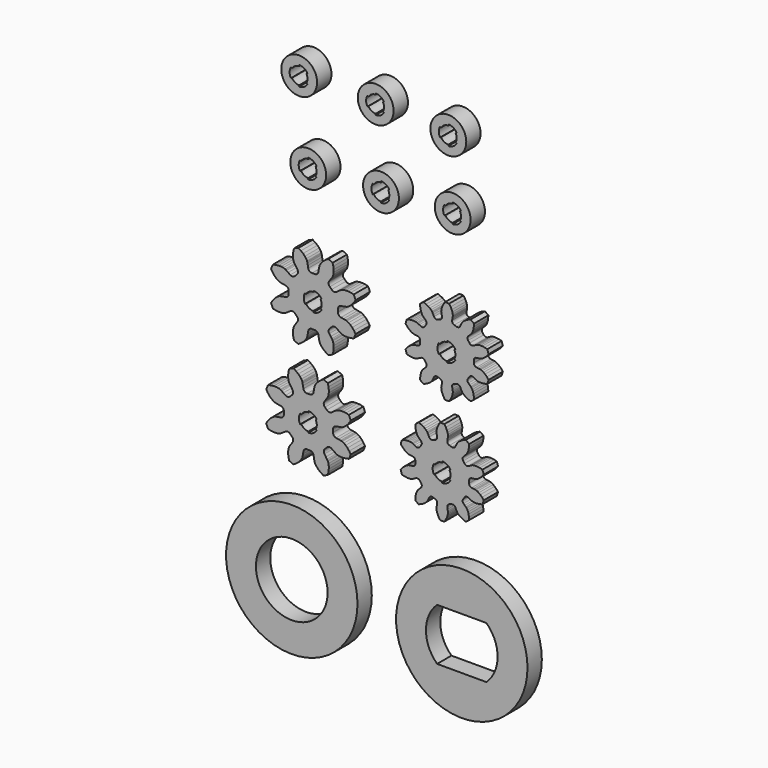
from build123d import *

# Parameters (mm, degrees)
F0_R     = 3
F1_DEPTH = 3
F0_R_2   = 11
F0_R_3   = 6


# Not quite as in the source:
# - ends of sketch curves that miss each other by under 0.0002 mm in the source are joined


with BuildPart() as f1:
    # F0 (on Front) → F1 (new body)
    with BuildSketch(Plane.XZ):
        with Locations((-0.182733, 41.3726)):
            Circle(F0_R)
        with BuildLine():
            ThreePointArc((-1.5683737345, 40.5726001533), (-1.782733, 41.3726), (-1.5683737345, 42.1725998467))
            Line((-1.5683737345, 42.1725998467), (-1.395169, 42.0726))
            ThreePointArc((-1.395169, 42.0726), (-0.8827330941, 42.585035511), (-0.182733, 42.7726))
            Line((-0.182733, 42.7726), (-0.182733, 42.9726))
            ThreePointArc((-0.182733, 42.9726), (0.6172670766, 42.7582406018), (1.2029077345, 42.1725998467))
            Line((1.2029077345, 42.1725998467), (1.029702, 42.0726))
            ThreePointArc((1.029702, 42.0726), (1.217267, 41.3726), (1.029702424, 40.6725997552))
            Line((1.029702424, 40.6725997552), (1.202908, 40.5726))
            ThreePointArc((1.202908, 40.5726), (0.6172670766, 39.9869593982), (-0.182733, 39.7726))
            Line((-0.182733, 39.7726), (-0.182733, 39.9726))
            ThreePointArc((-0.182733, 39.9726), (-0.8827330941, 40.160164489), (-1.395168674, 40.6726001882))
            Line((-1.395168674, 40.6726001882), (-1.5683737345, 40.5726001533))
        make_face(mode=Mode.SUBTRACT)
    extrude(amount=F1_DEPTH)


with BuildPart() as f1b:
    # F0 (on Front) → F1, piece 2 (new body)
    with BuildSketch(Plane.XZ):
        with Locations((12.707934, 29.490534)):
            Circle(F0_R)
        with BuildLine():
            ThreePointArc((11.3222932655, 28.6905341533), (11.107934, 29.490534), (11.3222932655, 30.2905338467))
            Line((11.3222932655, 30.2905338467), (11.495498, 30.190534))
            ThreePointArc((11.495498, 30.190534), (12.0079339059, 30.702969511), (12.707934, 30.890534))
            Line((12.707934, 30.890534), (12.707934, 31.090534))
            ThreePointArc((12.707934, 31.090534), (13.5079338601, 30.8761747268), (14.0935744845, 30.2905342798))
            Line((14.0935744845, 30.2905342798), (13.920369, 30.190534))
            ThreePointArc((13.920369, 30.190534), (14.107934, 29.490534), (13.920369424, 28.7905337552))
            Line((13.920369424, 28.7905337552), (14.093574, 28.690534))
            ThreePointArc((14.093574, 28.690534), (13.5079338601, 28.1048932732), (12.707934, 27.890534))
            Line((12.707934, 27.890534), (12.707934, 28.090534))
            ThreePointArc((12.707934, 28.090534), (12.0079339059, 28.278098489), (11.495498326, 28.7905341882))
            Line((11.495498326, 28.7905341882), (11.3222932655, 28.6905341533))
        make_face(mode=Mode.SUBTRACT)
    extrude(amount=F1_DEPTH)


with BuildPart() as f1c:
    # F0 (on Front) → F1, piece 3 (new body)
    with BuildSketch(Plane.XZ):
        with Locations((14.22888, -33.401225)):
            Circle(F0_R_2)
        with BuildLine():
            ThreePointArc((10.1003209518, -37.7549590508), (8.22888, -33.401225), (10.1003209518, -29.0474909492))
            Line((10.100321, -29.047491), (18.357439, -29.047491))
            ThreePointArc((18.3574390482, -29.0474909492), (20.22888, -33.401225), (18.3574390482, -37.7549590508))
            Line((18.357439, -37.754959), (10.100321, -37.754959))
        make_face(mode=Mode.SUBTRACT)
    extrude(amount=F1_DEPTH)


with BuildPart() as f1d:
    # F0 (on Front) → F1, piece 4 (new body)
    with BuildSketch(Plane.XZ):
        with BuildLine():
            ThreePointArc((13.143043773, -4.7593788891), (12.8821829065, -5.001442346), (12.5263362927, -5.0054792153))
            ThreePointArc((12.5263362927, -5.0054792153), (12.3443007022, -4.9419897506), (12.1597130423, -4.8863558479))
            ThreePointArc((12.1597130423, -4.8863558479), (11.8741990901, -4.6739288738), (11.8054388864, -4.32476498))
            Line((11.8054388864, -4.32476498), (11.855269, -4.040146))
            Line((11.855269, -4.040146), (11.893883, -3.81665))
            Line((11.893883, -3.81665), (11.91335, -3.700308))
            Line((11.91335, -3.700308), (11.920983, -3.648286))
            Line((11.920983, -3.648286), (11.923445, -3.579347))
            Line((11.923445, -3.579347), (11.903044, -3.355628))
            Line((11.903044, -3.355628), (11.840028, -3.082864))
            Line((11.840028, -3.082864), (11.732643, -2.782696))
            Line((11.732643, -2.782696), (11.549308, -2.410137))
            Line((11.549308, -2.410137), (11.30583, -2.030359))
            ThreePointArc((11.30583, -2.030359), (10.953724, -2.021744), (10.6016179893, -2.0303587818))
            Line((10.6016179893, -2.0303587818), (10.35814, -2.410137))
            Line((10.35814, -2.410137), (10.174805, -2.782696))
            Line((10.174805, -2.782696), (10.06742, -3.082864))
            Line((10.06742, -3.082864), (10.004404, -3.355628))
            Line((10.004404, -3.355628), (9.984003, -3.579347))
            Line((9.984003, -3.579347), (9.986465, -3.648286))
            Line((9.986465, -3.648286), (9.994098, -3.700308))
            Line((9.994098, -3.700308), (10.013565, -3.81665))
            Line((10.013565, -3.81665), (10.052179, -4.040146))
            Line((10.052179, -4.040146), (10.102009, -4.324765))
            ThreePointArc((10.102009, -4.324765), (10.0332489099, -4.6739288738), (9.7477349098, -4.8863556756))
            ThreePointArc((9.7477349098, -4.8863556756), (9.5631472978, -4.9419897506), (9.3811119632, -5.0054789014))
            ThreePointArc((9.3811119632, -5.0054789014), (9.0252650935, -5.001442346), (8.764404227, -4.7593788891))
            Line((8.764404227, -4.7593788891), (8.637422, -4.499829))
            Line((8.637422, -4.499829), (8.537294, -4.296319))
            Line((8.537294, -4.296319), (8.484659, -4.190755))
            Line((8.484659, -4.190755), (8.460257, -4.144181))
            Line((8.460257, -4.144181), (8.421727, -4.086962))
            Line((8.421727, -4.086962), (8.273723, -3.91796))
            Line((8.273723, -3.91796), (8.062416, -3.734329))
            Line((8.062416, -3.734329), (7.799105, -3.554608))
            Line((7.799105, -3.554608), (7.431799, -3.360962))
            Line((7.431799, -3.360962), (7.011593, -3.196829))
            ThreePointArc((7.011593, -3.196829), (6.7216698038, -3.3968219164), (6.4418739653, -3.6107539568))
            Line((6.4418739653, -3.6107539568), (6.468124, -4.061113))
            Line((6.468124, -4.061113), (6.538788, -4.470281))
            Line((6.538788, -4.470281), (6.628346, -4.776242))
            Line((6.628346, -4.776242), (6.737691, -5.033952))
            Line((6.737691, -5.033952), (6.852686, -5.226936))
            Line((6.852686, -5.226936), (6.895199, -5.281263))
            Line((6.895199, -5.281263), (6.931952, -5.318862))
            Line((6.931952, -5.318862), (7.016084, -5.401543))
            Line((7.016084, -5.401543), (7.178692, -5.559658))
            Line((7.178692, -5.559658), (7.3863, -5.76063))
            ThreePointArc((7.3863, -5.76063), (7.535905329, -6.0835261569), (7.4297816373, -6.423203712))
            ThreePointArc((7.4297816373, -6.423203712), (7.3131475737, -6.5767102981), (7.2031958069, -6.7350718719))
            ThreePointArc((7.2031958069, -6.7350718719), (6.912937393, -6.9409680096), (6.5596149724, -6.8984650521))
            Line((6.5596149724, -6.8984650521), (6.304324, -6.763122))
            Line((6.304324, -6.763122), (6.103699, -6.657333))
            Line((6.103699, -6.657333), (5.999067, -6.602868))
            Line((5.999067, -6.602868), (5.95195, -6.579533))
            Line((5.95195, -6.579533), (5.887146, -6.555888))
            Line((5.887146, -6.555888), (5.668072, -6.506157))
            Line((5.668072, -6.506157), (5.389185, -6.4818))
            Line((5.389185, -6.4818), (5.070524, -6.491173))
            Line((5.070524, -6.491173), (4.659546, -6.550407))
            Line((4.659546, -6.550407), (4.223117, -6.664611))
            ThreePointArc((4.223117, -6.664611), (4.106117181, -6.996821338), (4.0055036402, -7.3343559023))
            Line((4.0055036402, -7.3343559023), (4.291455, -7.683276))
            Line((4.291455, -7.683276), (4.589126, -7.972764))
            Line((4.589126, -7.972764), (4.841419, -8.167651))
            Line((4.841419, -8.167651), (5.08136, -8.311871))
            Line((5.08136, -8.311871), (5.287825, -8.400406))
            Line((5.287825, -8.400406), (5.354151, -8.419369))
            Line((5.354151, -8.419369), (5.405986, -8.428185))
            Line((5.405986, -8.428185), (5.522649, -8.445623))
            Line((5.522649, -8.445623), (5.747139, -8.477962))
            Line((5.747139, -8.477962), (6.033226, -8.518523))
            ThreePointArc((6.033226, -8.518523), (6.3440523322, -8.6918157461), (6.4578534569, -9.0289989767))
            ThreePointArc((6.4578534569, -9.0289989767), (6.453724, -9.221744), (6.4578537438, -9.414489011))
            ThreePointArc((6.4578537438, -9.414489011), (6.3440522875, -9.7516723076), (6.0332259646, -9.9249647496))
            Line((6.0332259646, -9.9249647496), (5.747139, -9.965526))
            Line((5.747139, -9.965526), (5.522649, -9.997865))
            Line((5.522649, -9.997865), (5.405986, -10.015303))
            Line((5.405986, -10.015303), (5.354151, -10.024119))
            Line((5.354151, -10.024119), (5.287825, -10.043082))
            Line((5.287825, -10.043082), (5.08136, -10.131617))
            Line((5.08136, -10.131617), (4.841419, -10.275837))
            Line((4.841419, -10.275837), (4.589126, -10.470724))
            Line((4.589126, -10.470724), (4.291455, -10.760212))
            Line((4.291455, -10.760212), (4.005504, -11.109132))
            ThreePointArc((4.005504, -11.109132), (4.1061173301, -11.4466671209), (4.2231169849, -11.7788770057))
            Line((4.2231169849, -11.7788770057), (4.659546, -11.893081))
            Line((4.659546, -11.893081), (5.070524, -11.952315))
            Line((5.070524, -11.952315), (5.389185, -11.961688))
            Line((5.389185, -11.961688), (5.668072, -11.937331))
            Line((5.668072, -11.937331), (5.887146, -11.8876))
            Line((5.887146, -11.8876), (5.95195, -11.863955))
            Line((5.95195, -11.863955), (5.999067, -11.84062))
            Line((5.999067, -11.84062), (6.103699, -11.786155))
            Line((6.103699, -11.786155), (6.304324, -11.680366))
            Line((6.304324, -11.680366), (6.559615, -11.545023))
            ThreePointArc((6.559615, -11.545023), (6.912937393, -11.5025199904), (7.2031960279, -11.7084159815))
            ThreePointArc((7.2031960279, -11.7084159815), (7.3131480487, -11.8667783558), (7.4297819085, -12.0202850727))
            ThreePointArc((7.4297819085, -12.0202850727), (7.5359052806, -12.3599625806), (7.3862996155, -12.6828576024))
            Line((7.3862996155, -12.6828576024), (7.178692, -12.88383))
            Line((7.178692, -12.88383), (7.016084, -13.041945))
            Line((7.016084, -13.041945), (6.931952, -13.124626))
            Line((6.931952, -13.124626), (6.895199, -13.162225))
            Line((6.895199, -13.162225), (6.852686, -13.216552))
            Line((6.852686, -13.216552), (6.737691, -13.409536))
            Line((6.737691, -13.409536), (6.628346, -13.667246))
            Line((6.628346, -13.667246), (6.538788, -13.973207))
            Line((6.538788, -13.973207), (6.468124, -14.382375))
            Line((6.468124, -14.382375), (6.441874, -14.832734))
            ThreePointArc((6.441874, -14.832734), (6.7216700253, -15.0466662445), (7.0115933661, -15.2466594405))
            Line((7.0115933661, -15.2466594405), (7.431799, -15.082526))
            Line((7.431799, -15.082526), (7.799105, -14.88888))
            Line((7.799105, -14.88888), (8.062416, -14.709159))
            Line((8.062416, -14.709159), (8.273723, -14.525528))
            Line((8.273723, -14.525528), (8.421727, -14.356526))
            Line((8.421727, -14.356526), (8.460257, -14.299307))
            Line((8.460257, -14.299307), (8.484659, -14.252733))
            Line((8.484659, -14.252733), (8.537294, -14.147169))
            Line((8.537294, -14.147169), (8.637422, -13.943659))
            Line((8.637422, -13.943659), (8.764404, -13.684109))
            ThreePointArc((8.764404, -13.684109), (9.0252648386, -13.4420457557), (9.3811120348, -13.4380089068))
            ThreePointArc((9.3811120348, -13.4380089068), (9.5631475914, -13.5014983448), (9.7477352159, -13.557132224))
            ThreePointArc((9.7477352159, -13.557132224), (10.0332489814, -13.7695592395), (10.1020091136, -14.11872302))
            Line((10.1020091136, -14.11872302), (10.052179, -14.403342))
            Line((10.052179, -14.403342), (10.013565, -14.626838))
            Line((10.013565, -14.626838), (9.994098, -14.74318))
            Line((9.994098, -14.74318), (9.986465, -14.795202))
            Line((9.986465, -14.795202), (9.984003, -14.864141))
            Line((9.984003, -14.864141), (10.004404, -15.08786))
            Line((10.004404, -15.08786), (10.06742, -15.360624))
            Line((10.06742, -15.360624), (10.174805, -15.660792))
            Line((10.174805, -15.660792), (10.35814, -16.033351))
            Line((10.35814, -16.033351), (10.601618, -16.413129))
            ThreePointArc((10.601618, -16.413129), (10.953724, -16.421744), (11.3058299618, -16.4131292206))
            Line((11.3058299618, -16.4131292206), (11.549308, -16.033351))
            Line((11.549308, -16.033351), (11.732643, -15.660792))
            Line((11.732643, -15.660792), (11.840028, -15.360624))
            Line((11.840028, -15.360624), (11.903044, -15.08786))
            Line((11.903044, -15.08786), (11.923445, -14.864141))
            Line((11.923445, -14.864141), (11.920983, -14.795202))
            Line((11.920983, -14.795202), (11.91335, -14.74318))
            Line((11.91335, -14.74318), (11.893883, -14.626838))
            Line((11.893883, -14.626838), (11.855269, -14.403342))
            Line((11.855269, -14.403342), (11.805439, -14.118723))
            ThreePointArc((11.805439, -14.118723), (11.8741990186, -13.7695592395), (12.159712832, -13.5571323962))
            ThreePointArc((12.159712832, -13.5571323962), (12.3443004086, -13.5014983448), (12.5263357093, -13.4380092207))
            ThreePointArc((12.5263357093, -13.4380092207), (12.8821831614, -13.4420457557), (13.1430441674, -13.6841099182))
            Line((13.1430441674, -13.6841099182), (13.270026, -13.943659))
            Line((13.270026, -13.943659), (13.370154, -14.147169))
            Line((13.370154, -14.147169), (13.422789, -14.252733))
            Line((13.422789, -14.252733), (13.447191, -14.299307))
            Line((13.447191, -14.299307), (13.485721, -14.356526))
            Line((13.485721, -14.356526), (13.633725, -14.525528))
            Line((13.633725, -14.525528), (13.845032, -14.709159))
            Line((13.845032, -14.709159), (14.108343, -14.88888))
            Line((14.108343, -14.88888), (14.475649, -15.082526))
            Line((14.475649, -15.082526), (14.895855, -15.246659))
            ThreePointArc((14.895855, -15.246659), (15.1857779747, -15.0466662445), (15.4655740347, -14.8327340432))
            Line((15.4655740347, -14.8327340432), (15.439324, -14.382375))
            Line((15.439324, -14.382375), (15.36866, -13.973207))
            Line((15.36866, -13.973207), (15.279102, -13.667246))
            Line((15.279102, -13.667246), (15.169757, -13.409536))
            Line((15.169757, -13.409536), (15.054762, -13.216552))
            Line((15.054762, -13.216552), (15.012249, -13.162225))
            Line((15.012249, -13.162225), (14.975496, -13.124626))
            Line((14.975496, -13.124626), (14.891364, -13.041945))
            Line((14.891364, -13.041945), (14.728756, -12.88383))
            Line((14.728756, -12.88383), (14.521148, -12.682858))
            ThreePointArc((14.521148, -12.682858), (14.3715427226, -12.359962629), (14.4776662624, -12.0202844143))
            ThreePointArc((14.4776662624, -12.0202844143), (14.594300134, -11.8667781042), (14.7042517326, -11.7084168227))
            ThreePointArc((14.7042517326, -11.7084168227), (14.994510607, -11.5025199904), (15.3478330276, -11.5450229479))
            Line((15.3478330276, -11.5450229479), (15.603124, -11.680366))
            Line((15.603124, -11.680366), (15.803749, -11.786155))
            Line((15.803749, -11.786155), (15.908381, -11.84062))
            Line((15.908381, -11.84062), (15.955498, -11.863955))
            Line((15.955498, -11.863955), (16.020302, -11.8876))
            Line((16.020302, -11.8876), (16.239376, -11.937331))
            Line((16.239376, -11.937331), (16.518263, -11.961688))
            Line((16.518263, -11.961688), (16.836924, -11.952315))
            Line((16.836924, -11.952315), (17.247902, -11.893081))
            Line((17.247902, -11.893081), (17.684331, -11.778877))
            ThreePointArc((17.684331, -11.778877), (17.8013307104, -11.4466669962), (17.9019441756, -11.1091327761))
            Line((17.9019441756, -11.1091327761), (17.615993, -10.760212))
            Line((17.615993, -10.760212), (17.318322, -10.470724))
            Line((17.318322, -10.470724), (17.066029, -10.275837))
            Line((17.066029, -10.275837), (16.826088, -10.131617))
            Line((16.826088, -10.131617), (16.619623, -10.043082))
            Line((16.619623, -10.043082), (16.553297, -10.024119))
            Line((16.553297, -10.024119), (16.501462, -10.015303))
            Line((16.501462, -10.015303), (16.384799, -9.997865))
            Line((16.384799, -9.997865), (16.160309, -9.965526))
            Line((16.160309, -9.965526), (15.874222, -9.924965))
            ThreePointArc((15.874222, -9.924965), (15.5633956988, -9.7516722911), (15.4495945449, -9.4144889805))
            ThreePointArc((15.4495945449, -9.4144889805), (15.453724, -9.221744), (15.4495942581, -9.0289990318))
            ThreePointArc((15.4495942581, -9.0289990318), (15.5633956541, -8.6918157626), (15.8742218969, -8.51852327))
            Line((15.8742218969, -8.51852327), (16.160309, -8.477962))
            Line((16.160309, -8.477962), (16.384799, -8.445623))
            Line((16.384799, -8.445623), (16.501462, -8.428185))
            Line((16.501462, -8.428185), (16.553297, -8.419369))
            Line((16.553297, -8.419369), (16.619623, -8.400406))
            Line((16.619623, -8.400406), (16.826088, -8.311871))
            Line((16.826088, -8.311871), (17.066029, -8.167651))
            Line((17.066029, -8.167651), (17.318322, -7.972764))
            Line((17.318322, -7.972764), (17.615993, -7.683276))
            Line((17.615993, -7.683276), (17.901944, -7.334356))
            ThreePointArc((17.901944, -7.334356), (17.8013308596, -6.9968214627), (17.6843310151, -6.6646109943))
            Line((17.6843310151, -6.6646109943), (17.247902, -6.550407))
            Line((17.247902, -6.550407), (16.836924, -6.491173))
            Line((16.836924, -6.491173), (16.518263, -6.4818))
            Line((16.518263, -6.4818), (16.239376, -6.506157))
            Line((16.239376, -6.506157), (16.020302, -6.555888))
            Line((16.020302, -6.555888), (15.955498, -6.579533))
            Line((15.955498, -6.579533), (15.908381, -6.602868))
            Line((15.908381, -6.602868), (15.803749, -6.657333))
            Line((15.803749, -6.657333), (15.603124, -6.763122))
            Line((15.603124, -6.763122), (15.347833, -6.898465))
            ThreePointArc((15.347833, -6.898465), (14.994510607, -6.9409680096), (14.7042519721, -6.7350720185))
            ThreePointArc((14.7042519721, -6.7350720185), (14.5943006091, -6.5767105497), (14.4776669653, -6.4232040276))
            ThreePointArc((14.4776669653, -6.4232040276), (14.3715426742, -6.0835261085), (14.5211484016, -5.7606303811))
            Line((14.5211484016, -5.7606303811), (14.728756, -5.559658))
            Line((14.728756, -5.559658), (14.891364, -5.401543))
            Line((14.891364, -5.401543), (14.975496, -5.318862))
            Line((14.975496, -5.318862), (15.012249, -5.281263))
            Line((15.012249, -5.281263), (15.054762, -5.226936))
            Line((15.054762, -5.226936), (15.169757, -5.033952))
            Line((15.169757, -5.033952), (15.279102, -4.776242))
            Line((15.279102, -4.776242), (15.36866, -4.470281))
            Line((15.36866, -4.470281), (15.439324, -4.061113))
            Line((15.439324, -4.061113), (15.465574, -3.610754))
            ThreePointArc((15.465574, -3.610754), (15.1857781962, -3.3968219164), (14.8958550921, -3.1968288593))
            Line((14.8958550921, -3.1968288593), (14.475649, -3.360962))
            Line((14.475649, -3.360962), (14.108343, -3.554608))
            Line((14.108343, -3.554608), (13.845032, -3.734329))
            Line((13.845032, -3.734329), (13.633725, -3.91796))
            Line((13.633725, -3.91796), (13.485721, -4.086962))
            Line((13.485721, -4.086962), (13.447191, -4.144181))
            Line((13.447191, -4.144181), (13.422789, -4.190755))
            Line((13.422789, -4.190755), (13.370154, -4.296319))
            Line((13.370154, -4.296319), (13.270026, -4.499829))
            Line((13.270026, -4.499829), (13.143043773, -4.7593788891))
        make_face()
        with BuildLine():
            ThreePointArc((9.5680835155, -10.0217442798), (9.353724, -9.221744), (9.5680835155, -8.4217437202))
            Line((9.5680835155, -8.4217437202), (9.741289, -8.521744))
            ThreePointArc((9.741289, -8.521744), (10.2537241224, -8.009308364), (10.953724, -7.821744))
            Line((10.953724, -7.821744), (10.953724, -7.621744))
            ThreePointArc((10.953724, -7.621744), (11.7537240766, -7.8361033982), (12.3393647345, -8.4217441533))
            Line((12.3393647345, -8.4217441533), (12.16616, -8.521744))
            ThreePointArc((12.16616, -8.521744), (12.353724, -9.221744), (12.166159674, -9.9217438118))
            Line((12.166159674, -9.9217438118), (12.339365, -10.021744))
            ThreePointArc((12.339365, -10.021744), (11.7537240766, -10.6073846018), (10.953724, -10.821744))
            Line((10.953724, -10.821744), (10.953724, -10.621744))
            ThreePointArc((10.953724, -10.621744), (10.2537241224, -10.434179636), (9.741288576, -9.9217442448))
            Line((9.741288576, -9.9217442448), (9.5680835155, -10.0217442798))
        make_face(mode=Mode.SUBTRACT)
    extrude(amount=F1_DEPTH)


with BuildPart() as f1e:
    # F0 (on Front) → F1, piece 5 (new body)
    with BuildSketch(Plane.XZ):
        with Locations((11.978656, 40.770012)):
            Circle(F0_R)
        with BuildLine():
            ThreePointArc((10.5930152655, 39.9700121533), (10.378656, 40.770012), (10.5930152655, 41.5700118467))
            Line((10.5930152655, 41.5700118467), (10.76622, 41.470012))
            ThreePointArc((10.76622, 41.470012), (11.2786559059, 41.982447511), (11.978656, 42.170012))
            Line((11.978656, 42.170012), (11.978656, 42.370012))
            ThreePointArc((11.978656, 42.370012), (12.7786560766, 42.1556526018), (13.3642967345, 41.5700118467))
            Line((13.3642967345, 41.5700118467), (13.191091, 41.470012))
            ThreePointArc((13.191091, 41.470012), (13.378656, 40.770012), (13.191091424, 40.0700117552))
            Line((13.191091424, 40.0700117552), (13.364297, 39.970012))
            ThreePointArc((13.364297, 39.970012), (12.7786560766, 39.3843713982), (11.978656, 39.170012))
            Line((11.978656, 39.170012), (11.978656, 39.370012))
            ThreePointArc((11.978656, 39.370012), (11.2786559059, 39.557576489), (10.766220326, 40.0700121882))
            Line((10.766220326, 40.0700121882), (10.5930152655, 39.9700121533))
        make_face(mode=Mode.SUBTRACT)
    extrude(amount=F1_DEPTH)


with BuildPart() as f1f:
    # F0 (on Front) → F1, piece 6 (new body)
    with BuildSketch(Plane.XZ):
        with BuildLine():
            Line((-4.705382, 7.712101), (-4.96919, 7.850628))
            Line((-4.96919, 7.850628), (-5.016148, 7.86832))
            Line((-5.016148, 7.86832), (-5.054828, 7.880652))
            Line((-5.054828, 7.880652), (-5.110027, 7.892802))
            Line((-5.110027, 7.892802), (-5.267232, 7.922637))
            Line((-5.267232, 7.922637), (-5.590275, 7.98214))
            Line((-5.590275, 7.98214), (-6.009857, 8.058547))
            ThreePointArc((-6.009857, 8.058547), (-6.3758616121, 8.27828494), (-6.5052699472, 8.6850989972))
            ThreePointArc((-6.5052699472, 8.6850989972), (-6.49946, 8.903954), (-6.5052698508, 9.1228090079))
            ThreePointArc((-6.5052698508, 9.1228090079), (-6.3758615567, 9.5296231301), (-6.0098568574, 9.7493612146))
            Line((-6.0098568574, 9.7493612146), (-5.590275, 9.825768))
            Line((-5.590275, 9.825768), (-5.267232, 9.885271))
            Line((-5.267232, 9.885271), (-5.110027, 9.915106))
            Line((-5.110027, 9.915106), (-5.054828, 9.927256))
            Line((-5.054828, 9.927256), (-5.016148, 9.939588))
            Line((-5.016148, 9.939588), (-4.96919, 9.95728))
            Line((-4.96919, 9.95728), (-4.705382, 10.095807))
            Line((-4.705382, 10.095807), (-4.408211, 10.317379))
            Line((-4.408211, 10.317379), (-4.106544, 10.612691))
            Line((-4.106544, 10.612691), (-3.816783, 10.974283))
            Line((-3.816783, 10.974283), (-3.5505, 11.39576))
            ThreePointArc((-3.5505, 11.39576), (-3.6953636243, 11.7740800279), (-3.8604425516, 12.1440262148))
            Line((-3.8604425516, 12.1440262148), (-4.346761, 12.253765))
            Line((-4.346761, 12.253765), (-4.807338, 12.304557))
            Line((-4.807338, 12.304557), (-5.229466, 12.300063))
            Line((-5.229466, 12.300063), (-5.596273, 12.246607))
            Line((-5.596273, 12.246607), (-5.880766, 12.15802))
            Line((-5.880766, 12.15802), (-5.926481, 12.137326))
            Line((-5.926481, 12.137326), (-5.962552, 12.118695))
            Line((-5.962552, 12.118695), (-6.010175, 12.088254))
            Line((-6.010175, 12.088254), (-6.142432, 11.99819))
            Line((-6.142432, 11.99819), (-6.412932, 11.811839))
            Line((-6.412932, 11.811839), (-6.76365, 11.569178))
            ThreePointArc((-6.76365, 11.569178), (-7.177832399, 11.4657525161), (-7.5569989389, 11.6619080549))
            ThreePointArc((-7.5569989389, 11.6619080549), (-7.7076450269, 11.8207699717), (-7.8665072327, 11.9714157412))
            ThreePointArc((-7.8665072327, 11.9714157412), (-8.0626615328, 12.3505820196), (-7.9592357689, 12.7647638399))
            Line((-7.9592357689, 12.7647638399), (-7.716575, 13.115482))
            Line((-7.716575, 13.115482), (-7.530224, 13.385982))
            Line((-7.530224, 13.385982), (-7.44016, 13.518239))
            Line((-7.44016, 13.518239), (-7.409719, 13.565862))
            Line((-7.409719, 13.565862), (-7.391088, 13.601933))
            Line((-7.391088, 13.601933), (-7.370394, 13.647648))
            Line((-7.370394, 13.647648), (-7.281807, 13.932141))
            Line((-7.281807, 13.932141), (-7.228351, 14.298948))
            Line((-7.228351, 14.298948), (-7.223857, 14.721076))
            Line((-7.223857, 14.721076), (-7.274649, 15.181653))
            Line((-7.274649, 15.181653), (-7.384388, 15.667972))
            ThreePointArc((-7.384388, 15.667972), (-7.7543343252, 15.833050522), (-8.13265416, 15.9779135458))
            Line((-8.13265416, 15.9779135458), (-8.554131, 15.711631))
            Line((-8.554131, 15.711631), (-8.915723, 15.42187))
            Line((-8.915723, 15.42187), (-9.211035, 15.120203))
            Line((-9.211035, 15.120203), (-9.432607, 14.823032))
            Line((-9.432607, 14.823032), (-9.571134, 14.559224))
            Line((-9.571134, 14.559224), (-9.588826, 14.512266))
            Line((-9.588826, 14.512266), (-9.601158, 14.473586))
            Line((-9.601158, 14.473586), (-9.613308, 14.418387))
            Line((-9.613308, 14.418387), (-9.643143, 14.261182))
            Line((-9.643143, 14.261182), (-9.702646, 13.938139))
            Line((-9.702646, 13.938139), (-9.779053, 13.518557))
            ThreePointArc((-9.779053, 13.518557), (-9.9987909608, 13.1525523715), (-10.4056050502, 13.0231440556))
            ThreePointArc((-10.4056050502, 13.0231440556), (-10.62446, 13.028954), (-10.8433149549, 13.023144152))
            ThreePointArc((-10.8433149549, 13.023144152), (-11.2501290392, 13.1525523715), (-11.4698671826, 13.5185569668))
            Line((-11.4698671826, 13.5185569668), (-11.546274, 13.938139))
            Line((-11.546274, 13.938139), (-11.605777, 14.261182))
            Line((-11.605777, 14.261182), (-11.635612, 14.418387))
            Line((-11.635612, 14.418387), (-11.647762, 14.473586))
            Line((-11.647762, 14.473586), (-11.660094, 14.512266))
            Line((-11.660094, 14.512266), (-11.677786, 14.559224))
            Line((-11.677786, 14.559224), (-11.816313, 14.823032))
            Line((-11.816313, 14.823032), (-12.037885, 15.120203))
            Line((-12.037885, 15.120203), (-12.333197, 15.42187))
            Line((-12.333197, 15.42187), (-12.694789, 15.711631))
            Line((-12.694789, 15.711631), (-13.116266, 15.977914))
            ThreePointArc((-13.116266, 15.977914), (-13.4945856748, 15.833050522), (-13.8645318252, 15.6679716351))
            Line((-13.8645318252, 15.6679716351), (-13.974271, 15.181653))
            Line((-13.974271, 15.181653), (-14.025063, 14.721076))
            Line((-14.025063, 14.721076), (-14.020569, 14.298948))
            Line((-14.020569, 14.298948), (-13.967113, 13.932141))
            Line((-13.967113, 13.932141), (-13.878526, 13.647648))
            Line((-13.878526, 13.647648), (-13.857832, 13.601933))
            Line((-13.857832, 13.601933), (-13.839201, 13.565862))
            Line((-13.839201, 13.565862), (-13.80876, 13.518239))
            Line((-13.80876, 13.518239), (-13.718696, 13.385982))
            Line((-13.718696, 13.385982), (-13.532345, 13.115482))
            Line((-13.532345, 13.115482), (-13.289684, 12.764764))
            ThreePointArc((-13.289684, 12.764764), (-13.1862585104, 12.3505816503), (-13.3824135578, 11.9714155081))
            ThreePointArc((-13.3824135578, 11.9714155081), (-13.5412754724, 11.8207694724), (-13.691921244, 11.6619073203))
            ThreePointArc((-13.691921244, 11.6619073203), (-14.071087933, 11.4657524773), (-14.485270308, 11.5691785553))
            Line((-14.485270308, 11.5691785553), (-14.835988, 11.811839))
            Line((-14.835988, 11.811839), (-15.106488, 11.99819))
            Line((-15.106488, 11.99819), (-15.238745, 12.088254))
            Line((-15.238745, 12.088254), (-15.286368, 12.118695))
            Line((-15.286368, 12.118695), (-15.322439, 12.137326))
            Line((-15.322439, 12.137326), (-15.368154, 12.15802))
            Line((-15.368154, 12.15802), (-15.652647, 12.246607))
            Line((-15.652647, 12.246607), (-16.019454, 12.300063))
            Line((-16.019454, 12.300063), (-16.441582, 12.304557))
            Line((-16.441582, 12.304557), (-16.902159, 12.253765))
            Line((-16.902159, 12.253765), (-17.388478, 12.144026))
            ThreePointArc((-17.388478, 12.144026), (-17.553556522, 11.7740796748), (-17.6984195458, 11.39575984))
            Line((-17.6984195458, 11.39575984), (-17.432137, 10.974283))
            Line((-17.432137, 10.974283), (-17.142376, 10.612691))
            Line((-17.142376, 10.612691), (-16.840709, 10.317379))
            Line((-16.840709, 10.317379), (-16.543538, 10.095807))
            Line((-16.543538, 10.095807), (-16.27973, 9.95728))
            Line((-16.27973, 9.95728), (-16.232772, 9.939588))
            Line((-16.232772, 9.939588), (-16.194092, 9.927256))
            Line((-16.194092, 9.927256), (-16.138893, 9.915106))
            Line((-16.138893, 9.915106), (-15.981688, 9.885271))
            Line((-15.981688, 9.885271), (-15.658645, 9.825768))
            Line((-15.658645, 9.825768), (-15.239063, 9.749361))
            ThreePointArc((-15.239063, 9.749361), (-14.8730584433, 9.5296231301), (-14.7436500528, 9.1228090028))
            ThreePointArc((-14.7436500528, 9.1228090028), (-14.74946, 8.903954), (-14.7436501492, 8.6850989921))
            ThreePointArc((-14.7436501492, 8.6850989921), (-14.8730583879, 8.27828494), (-15.2390629668, 8.0585468174))
            Line((-15.2390629668, 8.0585468174), (-15.658645, 7.98214))
            Line((-15.658645, 7.98214), (-15.981688, 7.922637))
            Line((-15.981688, 7.922637), (-16.138893, 7.892802))
            Line((-16.138893, 7.892802), (-16.194092, 7.880652))
            Line((-16.194092, 7.880652), (-16.232772, 7.86832))
            Line((-16.232772, 7.86832), (-16.27973, 7.850628))
            Line((-16.27973, 7.850628), (-16.543538, 7.712101))
            Line((-16.543538, 7.712101), (-16.840709, 7.490529))
            Line((-16.840709, 7.490529), (-17.142376, 7.195217))
            Line((-17.142376, 7.195217), (-17.432137, 6.833625))
            Line((-17.432137, 6.833625), (-17.69842, 6.412148))
            ThreePointArc((-17.69842, 6.412148), (-17.553556875, 6.0338291775), (-17.3884780247, 5.6638829882))
            Line((-17.3884780247, 5.6638829882), (-16.902159, 5.554143))
            Line((-16.902159, 5.554143), (-16.441582, 5.503351))
            Line((-16.441582, 5.503351), (-16.019454, 5.507845))
            Line((-16.019454, 5.507845), (-15.652647, 5.561301))
            Line((-15.652647, 5.561301), (-15.368154, 5.649888))
            Line((-15.368154, 5.649888), (-15.322439, 5.670582))
            Line((-15.322439, 5.670582), (-15.286368, 5.689213))
            Line((-15.286368, 5.689213), (-15.238745, 5.719654))
            Line((-15.238745, 5.719654), (-15.106488, 5.809718))
            Line((-15.106488, 5.809718), (-14.835988, 5.996069))
            Line((-14.835988, 5.996069), (-14.48527, 6.23873))
            ThreePointArc((-14.48527, 6.23873), (-14.0710880196, 6.3421555328), (-13.6919220053, 6.1460009952))
            ThreePointArc((-13.6919220053, 6.1460009952), (-13.5412759717, 5.9871390269), (-13.3824138174, 5.836493203))
            ThreePointArc((-13.3824138174, 5.836493203), (-13.1862585969, 5.45732709), (-13.289683763, 5.0431448359))
            Line((-13.289683763, 5.0431448359), (-13.532345, 4.692426))
            Line((-13.532345, 4.692426), (-13.718696, 4.421926))
            Line((-13.718696, 4.421926), (-13.80876, 4.289669))
            Line((-13.80876, 4.289669), (-13.839201, 4.242046))
            Line((-13.839201, 4.242046), (-13.857832, 4.205975))
            Line((-13.857832, 4.205975), (-13.878526, 4.16026))
            Line((-13.878526, 4.16026), (-13.967113, 3.875767))
            Line((-13.967113, 3.875767), (-14.020569, 3.50896))
            Line((-14.020569, 3.50896), (-14.025063, 3.086832))
            Line((-14.025063, 3.086832), (-13.974271, 2.626255))
            Line((-13.974271, 2.626255), (-13.864532, 2.139936))
            ThreePointArc((-13.864532, 2.139936), (-13.4945860279, 1.9748576243), (-13.1162661534, 1.8299945646))
            Line((-13.1162661534, 1.8299945646), (-12.694789, 2.096277))
            Line((-12.694789, 2.096277), (-12.333197, 2.386038))
            Line((-12.333197, 2.386038), (-12.037885, 2.687705))
            Line((-12.037885, 2.687705), (-11.816313, 2.984876))
            Line((-11.816313, 2.984876), (-11.677786, 3.248684))
            Line((-11.677786, 3.248684), (-11.660094, 3.295642))
            Line((-11.660094, 3.295642), (-11.647762, 3.334322))
            Line((-11.647762, 3.334322), (-11.635612, 3.389521))
            Line((-11.635612, 3.389521), (-11.605777, 3.546726))
            Line((-11.605777, 3.546726), (-11.546274, 3.869769))
            Line((-11.546274, 3.869769), (-11.469867, 4.289351))
            ThreePointArc((-11.469867, 4.289351), (-11.2501286741, 4.6553559172), (-10.8433150028, 4.7847639472))
            ThreePointArc((-10.8433150028, 4.7847639472), (-10.62446, 4.778954), (-10.4056049921, 4.7847638508))
            ThreePointArc((-10.4056049921, 4.7847638508), (-9.9987913259, 4.6553559172), (-9.7790529932, 4.2893520012))
            Line((-9.7790529932, 4.2893520012), (-9.702646, 3.869769))
            Line((-9.702646, 3.869769), (-9.643143, 3.546726))
            Line((-9.643143, 3.546726), (-9.613308, 3.389521))
            Line((-9.613308, 3.389521), (-9.601158, 3.334322))
            Line((-9.601158, 3.334322), (-9.588826, 3.295642))
            Line((-9.588826, 3.295642), (-9.571134, 3.248684))
            Line((-9.571134, 3.248684), (-9.432607, 2.984876))
            Line((-9.432607, 2.984876), (-9.211035, 2.687705))
            Line((-9.211035, 2.687705), (-8.915723, 2.386038))
            Line((-8.915723, 2.386038), (-8.554131, 2.096277))
            Line((-8.554131, 2.096277), (-8.132654, 1.829994))
            ThreePointArc((-8.132654, 1.829994), (-7.7543339721, 1.9748576243), (-7.3843877852, 2.1399365516))
            Line((-7.3843877852, 2.1399365516), (-7.274649, 2.626255))
            Line((-7.274649, 2.626255), (-7.223857, 3.086832))
            Line((-7.223857, 3.086832), (-7.228351, 3.50896))
            Line((-7.228351, 3.50896), (-7.281807, 3.875767))
            Line((-7.281807, 3.875767), (-7.370394, 4.16026))
            Line((-7.370394, 4.16026), (-7.391088, 4.205975))
            Line((-7.391088, 4.205975), (-7.409719, 4.242046))
            Line((-7.409719, 4.242046), (-7.44016, 4.289669))
            Line((-7.44016, 4.289669), (-7.530224, 4.421926))
            Line((-7.530224, 4.421926), (-7.716575, 4.692426))
            Line((-7.716575, 4.692426), (-7.959236, 5.043144))
            ThreePointArc((-7.959236, 5.043144), (-8.0626614463, 5.4573267207), (-7.866506498, 5.8364924417))
            ThreePointArc((-7.866506498, 5.8364924417), (-7.7076445276, 5.9871385276), (-7.5569987059, 6.1460007355))
            ThreePointArc((-7.5569987059, 6.1460007355), (-7.1778323125, 6.342155494), (-6.7636501601, 6.2387297689))
            Line((-6.7636501601, 6.2387297689), (-6.412932, 5.996069))
            Line((-6.412932, 5.996069), (-6.142432, 5.809718))
            Line((-6.142432, 5.809718), (-6.010175, 5.719654))
            Line((-6.010175, 5.719654), (-5.962552, 5.689213))
            Line((-5.962552, 5.689213), (-5.926481, 5.670582))
            Line((-5.926481, 5.670582), (-5.880766, 5.649888))
            Line((-5.880766, 5.649888), (-5.596273, 5.561301))
            Line((-5.596273, 5.561301), (-5.229466, 5.507845))
            Line((-5.229466, 5.507845), (-4.807338, 5.503351))
            Line((-4.807338, 5.503351), (-4.346761, 5.554143))
            Line((-4.346761, 5.554143), (-3.860442, 5.663882))
            ThreePointArc((-3.860442, 5.663882), (-3.6953632712, 6.0338288245), (-3.5505002512, 6.4121487362))
            Line((-3.5505002512, 6.4121487362), (-3.816783, 6.833625))
            Line((-3.816783, 6.833625), (-4.106544, 7.195217))
            Line((-4.106544, 7.195217), (-4.408211, 7.490529))
            Line((-4.408211, 7.490529), (-4.705382, 7.712101))
        make_face()
        with BuildLine():
            ThreePointArc((-9.2388195155, 8.1039537202), (-9.8244601399, 7.5183132732), (-10.62446, 7.303954))
            Line((-10.62446, 7.303954), (-10.62446, 7.503954))
            ThreePointArc((-10.62446, 7.503954), (-11.3244600941, 7.691518489), (-11.836895674, 8.2039541882))
            Line((-11.836895674, 8.2039541882), (-12.010101, 8.103954))
            ThreePointArc((-12.010101, 8.103954), (-12.22446, 8.903954), (-12.0101007345, 9.7039538467))
            Line((-12.0101007345, 9.7039538467), (-11.836896, 9.603954))
            ThreePointArc((-11.836896, 9.603954), (-11.3244600941, 10.116389511), (-10.62446, 10.303954))
            Line((-10.62446, 10.303954), (-10.62446, 10.503954))
            ThreePointArc((-10.62446, 10.503954), (-9.8244601399, 10.2895947268), (-9.2388195155, 9.7039542798))
            Line((-9.2388195155, 9.7039542798), (-9.412025, 9.603954))
            ThreePointArc((-9.412025, 9.603954), (-9.22446, 8.903954), (-9.412024576, 8.2039537552))
            Line((-9.412024576, 8.2039537552), (-9.2388195155, 8.1039537202))
        make_face(mode=Mode.SUBTRACT)
    extrude(amount=F1_DEPTH)


with BuildPart() as f1g:
    # F0 (on Front) → F1, piece 7 (new body)
    with BuildSketch(Plane.XZ):
        with Locations((0.703662, 28.726432)):
            Circle(F0_R)
        with BuildLine():
            ThreePointArc((-0.6819784845, 27.9264317202), (-0.896338, 28.726432), (-0.6819784845, 29.5264322798))
            Line((-0.6819784845, 29.5264322798), (-0.508773, 29.426432))
            ThreePointArc((-0.508773, 29.426432), (0.0036621224, 29.938867636), (0.703662, 30.126432))
            Line((0.703662, 30.126432), (0.703662, 30.326432))
            ThreePointArc((0.703662, 30.326432), (1.5036620766, 30.1120726018), (2.0893027345, 29.5264318467))
            Line((2.0893027345, 29.5264318467), (1.916098, 29.426432))
            ThreePointArc((1.916098, 29.426432), (2.103662, 28.726432), (1.916097674, 28.0264321882))
            Line((1.916097674, 28.0264321882), (2.089303, 27.926432))
            ThreePointArc((2.089303, 27.926432), (1.5036620766, 27.3407913982), (0.703662, 27.126432))
            Line((0.703662, 27.126432), (0.703662, 27.326432))
            ThreePointArc((0.703662, 27.326432), (0.0036621224, 27.513996364), (-0.508773424, 28.0264317552))
            Line((-0.508773424, 28.0264317552), (-0.6819784845, 27.9264317202))
        make_face(mode=Mode.SUBTRACT)
    extrude(amount=F1_DEPTH)


with BuildPart() as f1h:
    # F0 (on Front) → F1, piece 8 (new body)
    with BuildSketch(Plane.XZ):
        with BuildLine():
            ThreePointArc((12.9679670902, 13.1219433244), (12.6824530901, 13.3343701262), (12.6136928864, 13.68353402))
            Line((12.6136928864, 13.68353402), (12.663523, 13.968153))
            Line((12.663523, 13.968153), (12.702137, 14.191649))
            Line((12.702137, 14.191649), (12.721604, 14.307991))
            Line((12.721604, 14.307991), (12.729237, 14.360013))
            Line((12.729237, 14.360013), (12.731699, 14.428952))
            Line((12.731699, 14.428952), (12.711298, 14.652671))
            Line((12.711298, 14.652671), (12.648282, 14.925435))
            Line((12.648282, 14.925435), (12.540897, 15.225603))
            Line((12.540897, 15.225603), (12.357562, 15.598162))
            Line((12.357562, 15.598162), (12.114084, 15.97794))
            ThreePointArc((12.114084, 15.97794), (11.761978, 15.986555), (11.4098719893, 15.9779402182))
            Line((11.4098719893, 15.9779402182), (11.166394, 15.598162))
            Line((11.166394, 15.598162), (10.983059, 15.225603))
            Line((10.983059, 15.225603), (10.875674, 14.925435))
            Line((10.875674, 14.925435), (10.812658, 14.652671))
            Line((10.812658, 14.652671), (10.792257, 14.428952))
            Line((10.792257, 14.428952), (10.794719, 14.360013))
            Line((10.794719, 14.360013), (10.802352, 14.307991))
            Line((10.802352, 14.307991), (10.821819, 14.191649))
            Line((10.821819, 14.191649), (10.860433, 13.968153))
            Line((10.860433, 13.968153), (10.910263, 13.683534))
            ThreePointArc((10.910263, 13.683534), (10.8415029099, 13.3343701262), (10.5559889098, 13.1219433244))
            ThreePointArc((10.5559889098, 13.1219433244), (10.3714012978, 13.0663092494), (10.1893659632, 13.0028200986))
            ThreePointArc((10.1893659632, 13.0028200986), (9.8335192558, 13.0068565892), (9.572658227, 13.2489201109))
            Line((9.572658227, 13.2489201109), (9.445676, 13.50847))
            Line((9.445676, 13.50847), (9.345548, 13.71198))
            Line((9.345548, 13.71198), (9.292913, 13.817544))
            Line((9.292913, 13.817544), (9.268511, 13.864118))
            Line((9.268511, 13.864118), (9.229981, 13.921337))
            Line((9.229981, 13.921337), (9.081977, 14.090339))
            Line((9.081977, 14.090339), (8.87067, 14.27397))
            Line((8.87067, 14.27397), (8.607359, 14.453691))
            Line((8.607359, 14.453691), (8.240053, 14.647337))
            Line((8.240053, 14.647337), (7.819847, 14.81147))
            ThreePointArc((7.819847, 14.81147), (7.5299238038, 14.6114770836), (7.2501279653, 14.3975450432))
            Line((7.2501279653, 14.3975450432), (7.276378, 13.947186))
            Line((7.276378, 13.947186), (7.347042, 13.538018))
            Line((7.347042, 13.538018), (7.4366, 13.232057))
            Line((7.4366, 13.232057), (7.545945, 12.974347))
            Line((7.545945, 12.974347), (7.66094, 12.781363))
            Line((7.66094, 12.781363), (7.703453, 12.727036))
            Line((7.703453, 12.727036), (7.740206, 12.689437))
            Line((7.740206, 12.689437), (7.824338, 12.606756))
            Line((7.824338, 12.606756), (7.986946, 12.448641))
            Line((7.986946, 12.448641), (8.194554, 12.247669))
            ThreePointArc((8.194554, 12.247669), (8.344159329, 11.9247728431), (8.2380356373, 11.585095288))
            ThreePointArc((8.2380356373, 11.585095288), (8.1214015737, 11.4315887019), (8.0114498069, 11.2732271281))
            ThreePointArc((8.0114498069, 11.2732271281), (7.721191393, 11.0673309904), (7.3678689724, 11.1098339479))
            Line((7.3678689724, 11.1098339479), (7.112578, 11.245177))
            Line((7.112578, 11.245177), (6.911953, 11.350966))
            Line((6.911953, 11.350966), (6.807321, 11.405431))
            Line((6.807321, 11.405431), (6.760204, 11.428766))
            Line((6.760204, 11.428766), (6.6954, 11.452411))
            Line((6.6954, 11.452411), (6.476326, 11.502142))
            Line((6.476326, 11.502142), (6.197439, 11.526499))
            Line((6.197439, 11.526499), (5.878778, 11.517126))
            Line((5.878778, 11.517126), (5.4678, 11.457892))
            Line((5.4678, 11.457892), (5.031371, 11.343688))
            ThreePointArc((5.031371, 11.343688), (4.914371181, 11.011477662), (4.8137576402, 10.6739430977))
            Line((4.8137576402, 10.6739430977), (5.099709, 10.325023))
            Line((5.099709, 10.325023), (5.39738, 10.035535))
            Line((5.39738, 10.035535), (5.649673, 9.840648))
            Line((5.649673, 9.840648), (5.889614, 9.696428))
            Line((5.889614, 9.696428), (6.096079, 9.607893))
            Line((6.096079, 9.607893), (6.162405, 9.58893))
            Line((6.162405, 9.58893), (6.21424, 9.580114))
            Line((6.21424, 9.580114), (6.330903, 9.562676))
            Line((6.330903, 9.562676), (6.555393, 9.530337))
            Line((6.555393, 9.530337), (6.84148, 9.489776))
            ThreePointArc((6.84148, 9.489776), (7.1523063322, 9.3164832539), (7.2661074569, 8.9793000233))
            ThreePointArc((7.2661074569, 8.9793000233), (7.261978, 8.786555), (7.2661077438, 8.593809989))
            ThreePointArc((7.2661077438, 8.593809989), (7.1523062875, 8.2566266924), (6.8414799646, 8.0833342504))
            Line((6.8414799646, 8.0833342504), (6.555393, 8.042773))
            Line((6.555393, 8.042773), (6.330903, 8.010434))
            Line((6.330903, 8.010434), (6.21424, 7.992996))
            Line((6.21424, 7.992996), (6.162405, 7.98418))
            Line((6.162405, 7.98418), (6.096079, 7.965217))
            Line((6.096079, 7.965217), (5.889614, 7.876682))
            Line((5.889614, 7.876682), (5.649673, 7.732462))
            Line((5.649673, 7.732462), (5.39738, 7.537575))
            Line((5.39738, 7.537575), (5.099709, 7.248087))
            Line((5.099709, 7.248087), (4.813758, 6.899167))
            ThreePointArc((4.813758, 6.899167), (4.914371181, 6.561632338), (5.0313709849, 6.2294219943))
            Line((5.0313709849, 6.2294219943), (5.4678, 6.115218))
            Line((5.4678, 6.115218), (5.878778, 6.055984))
            Line((5.878778, 6.055984), (6.197439, 6.046611))
            Line((6.197439, 6.046611), (6.476326, 6.070968))
            Line((6.476326, 6.070968), (6.6954, 6.120699))
            Line((6.6954, 6.120699), (6.760204, 6.144344))
            Line((6.760204, 6.144344), (6.807321, 6.167679))
            Line((6.807321, 6.167679), (6.911953, 6.222144))
            Line((6.911953, 6.222144), (7.112578, 6.327933))
            Line((7.112578, 6.327933), (7.367869, 6.463276))
            ThreePointArc((7.367869, 6.463276), (7.721191393, 6.5057790096), (8.0114500279, 6.2998830185))
            ThreePointArc((8.0114500279, 6.2998830185), (8.1214018038, 6.1415209814), (8.2380359085, 5.9880139273))
            ThreePointArc((8.2380359085, 5.9880139273), (8.3441592806, 5.6483364194), (8.1945536155, 5.3254413976))
            Line((8.1945536155, 5.3254413976), (7.986946, 5.124469))
            Line((7.986946, 5.124469), (7.824338, 4.966354))
            Line((7.824338, 4.966354), (7.740206, 4.883673))
            Line((7.740206, 4.883673), (7.703453, 4.846074))
            Line((7.703453, 4.846074), (7.66094, 4.791747))
            Line((7.66094, 4.791747), (7.545945, 4.598763))
            Line((7.545945, 4.598763), (7.4366, 4.341053))
            Line((7.4366, 4.341053), (7.347042, 4.035092))
            Line((7.347042, 4.035092), (7.276378, 3.625924))
            Line((7.276378, 3.625924), (7.250128, 3.175565))
            ThreePointArc((7.250128, 3.175565), (7.5299238038, 2.9616329164), (7.8198469079, 2.7616398593))
            Line((7.8198469079, 2.7616398593), (8.240053, 2.925773))
            Line((8.240053, 2.925773), (8.607359, 3.119419))
            Line((8.607359, 3.119419), (8.87067, 3.29914))
            Line((8.87067, 3.29914), (9.081977, 3.482771))
            Line((9.081977, 3.482771), (9.229981, 3.651773))
            Line((9.229981, 3.651773), (9.268511, 3.708992))
            Line((9.268511, 3.708992), (9.292913, 3.755566))
            Line((9.292913, 3.755566), (9.345548, 3.86113))
            Line((9.345548, 3.86113), (9.445676, 4.06464))
            Line((9.445676, 4.06464), (9.572658, 4.32419))
            ThreePointArc((9.572658, 4.32419), (9.8335192558, 4.5662534108), (10.1893660348, 4.5702900932))
            ThreePointArc((10.1893660348, 4.5702900932), (10.3714012978, 4.5068007506), (10.5559889577, 4.4511668479))
            ThreePointArc((10.5559889577, 4.4511668479), (10.8415029814, 4.2387397605), (10.9102631136, 3.88957598))
            Line((10.9102631136, 3.88957598), (10.860433, 3.604957))
            Line((10.860433, 3.604957), (10.821819, 3.381461))
            Line((10.821819, 3.381461), (10.802352, 3.265119))
            Line((10.802352, 3.265119), (10.794719, 3.213097))
            Line((10.794719, 3.213097), (10.792257, 3.144158))
            Line((10.792257, 3.144158), (10.812658, 2.920439))
            Line((10.812658, 2.920439), (10.875674, 2.647675))
            Line((10.875674, 2.647675), (10.983059, 2.347507))
            Line((10.983059, 2.347507), (11.166394, 1.974948))
            Line((11.166394, 1.974948), (11.409872, 1.59517))
            ThreePointArc((11.409872, 1.59517), (11.761978, 1.586555), (12.1140840107, 1.5951697818))
            Line((12.1140840107, 1.5951697818), (12.357562, 1.974948))
            Line((12.357562, 1.974948), (12.540897, 2.347507))
            Line((12.540897, 2.347507), (12.648282, 2.647675))
            Line((12.648282, 2.647675), (12.711298, 2.920439))
            Line((12.711298, 2.920439), (12.731699, 3.144158))
            Line((12.731699, 3.144158), (12.729237, 3.213097))
            Line((12.729237, 3.213097), (12.721604, 3.265119))
            Line((12.721604, 3.265119), (12.702137, 3.381461))
            Line((12.702137, 3.381461), (12.663523, 3.604957))
            Line((12.663523, 3.604957), (12.613693, 3.889576))
            ThreePointArc((12.613693, 3.889576), (12.6824530186, 4.2387397605), (12.967966832, 4.4511666038))
            ThreePointArc((12.967966832, 4.4511666038), (13.1525547022, 4.5068007506), (13.3345900368, 4.5702899014))
            ThreePointArc((13.3345900368, 4.5702899014), (13.6904367442, 4.5662534108), (13.951297773, 4.3241898891))
            Line((13.951297773, 4.3241898891), (14.07828, 4.06464))
            Line((14.07828, 4.06464), (14.178408, 3.86113))
            Line((14.178408, 3.86113), (14.231043, 3.755566))
            Line((14.231043, 3.755566), (14.255445, 3.708992))
            Line((14.255445, 3.708992), (14.293975, 3.651773))
            Line((14.293975, 3.651773), (14.441979, 3.482771))
            Line((14.441979, 3.482771), (14.653286, 3.29914))
            Line((14.653286, 3.29914), (14.916597, 3.119419))
            Line((14.916597, 3.119419), (15.283903, 2.925773))
            Line((15.283903, 2.925773), (15.704109, 2.76164))
            ThreePointArc((15.704109, 2.76164), (15.9940321962, 2.9616329164), (16.2738280347, 3.1755649568))
            Line((16.2738280347, 3.1755649568), (16.247578, 3.625924))
            Line((16.247578, 3.625924), (16.176914, 4.035092))
            Line((16.176914, 4.035092), (16.087356, 4.341053))
            Line((16.087356, 4.341053), (15.978011, 4.598763))
            Line((15.978011, 4.598763), (15.863016, 4.791747))
            Line((15.863016, 4.791747), (15.820503, 4.846074))
            Line((15.820503, 4.846074), (15.78375, 4.883673))
            Line((15.78375, 4.883673), (15.699618, 4.966354))
            Line((15.699618, 4.966354), (15.53701, 5.124469))
            Line((15.53701, 5.124469), (15.329402, 5.325441))
            ThreePointArc((15.329402, 5.325441), (15.1797967429, 5.6483360607), (15.2859198757, 5.9880140987))
            ThreePointArc((15.2859198757, 5.9880140987), (15.402554379, 6.1415212329), (15.5125061931, 6.2998828719))
            ThreePointArc((15.5125061931, 6.2998828719), (15.802764607, 6.5057790096), (16.1560870276, 6.4632760521))
            Line((16.1560870276, 6.4632760521), (16.411378, 6.327933))
            Line((16.411378, 6.327933), (16.612003, 6.222144))
            Line((16.612003, 6.222144), (16.716635, 6.167679))
            Line((16.716635, 6.167679), (16.763752, 6.144344))
            Line((16.763752, 6.144344), (16.828556, 6.120699))
            Line((16.828556, 6.120699), (17.04763, 6.070968))
            Line((17.04763, 6.070968), (17.326517, 6.046611))
            Line((17.326517, 6.046611), (17.645178, 6.055984))
            Line((17.645178, 6.055984), (18.056156, 6.115218))
            Line((18.056156, 6.115218), (18.492585, 6.229422))
            ThreePointArc((18.492585, 6.229422), (18.609584819, 6.561632338), (18.7101983598, 6.8991669023))
            Line((18.7101983598, 6.8991669023), (18.424247, 7.248087))
            Line((18.424247, 7.248087), (18.126576, 7.537575))
            Line((18.126576, 7.537575), (17.874283, 7.732462))
            Line((17.874283, 7.732462), (17.634342, 7.876682))
            Line((17.634342, 7.876682), (17.427877, 7.965217))
            Line((17.427877, 7.965217), (17.361551, 7.98418))
            Line((17.361551, 7.98418), (17.309716, 7.992996))
            Line((17.309716, 7.992996), (17.193053, 8.010434))
            Line((17.193053, 8.010434), (16.968563, 8.042773))
            Line((16.968563, 8.042773), (16.682476, 8.083334))
            ThreePointArc((16.682476, 8.083334), (16.3716496988, 8.2566267089), (16.2578485449, 8.5938100195))
            ThreePointArc((16.2578485449, 8.5938100195), (16.261978, 8.786555), (16.2578482562, 8.979300011))
            ThreePointArc((16.2578482562, 8.979300011), (16.3716496541, 9.3164832374), (16.6824758969, 9.48977573))
            Line((16.6824758969, 9.48977573), (16.968563, 9.530337))
            Line((16.968563, 9.530337), (17.193053, 9.562676))
            Line((17.193053, 9.562676), (17.309716, 9.580114))
            Line((17.309716, 9.580114), (17.361551, 9.58893))
            Line((17.361551, 9.58893), (17.427877, 9.607893))
            Line((17.427877, 9.607893), (17.634342, 9.696428))
            Line((17.634342, 9.696428), (17.874283, 9.840648))
            Line((17.874283, 9.840648), (18.126576, 10.035535))
            Line((18.126576, 10.035535), (18.424247, 10.325023))
            Line((18.424247, 10.325023), (18.710198, 10.673943))
            ThreePointArc((18.710198, 10.673943), (18.609584819, 11.011477662), (18.4925850151, 11.3436880057))
            Line((18.4925850151, 11.3436880057), (18.056156, 11.457892))
            Line((18.056156, 11.457892), (17.645178, 11.517126))
            Line((17.645178, 11.517126), (17.326517, 11.526499))
            Line((17.326517, 11.526499), (17.04763, 11.502142))
            Line((17.04763, 11.502142), (16.828556, 11.452411))
            Line((16.828556, 11.452411), (16.763752, 11.428766))
            Line((16.763752, 11.428766), (16.716635, 11.405431))
            Line((16.716635, 11.405431), (16.612003, 11.350966))
            Line((16.612003, 11.350966), (16.411378, 11.245177))
            Line((16.411378, 11.245177), (16.156087, 11.109834))
            ThreePointArc((16.156087, 11.109834), (15.802764607, 11.0673309904), (15.5125059721, 11.2732269815))
            ThreePointArc((15.5125059721, 11.2732269815), (15.4025546091, 11.4315884503), (15.2859209653, 11.5850949724))
            ThreePointArc((15.2859209653, 11.5850949724), (15.1797966945, 11.9247732017), (15.3294024016, 12.2476686189))
            Line((15.3294024016, 12.2476686189), (15.53701, 12.448641))
            Line((15.53701, 12.448641), (15.699618, 12.606756))
            Line((15.699618, 12.606756), (15.78375, 12.689437))
            Line((15.78375, 12.689437), (15.820503, 12.727036))
            Line((15.820503, 12.727036), (15.863016, 12.781363))
            Line((15.863016, 12.781363), (15.978011, 12.974347))
            Line((15.978011, 12.974347), (16.087356, 13.232057))
            Line((16.087356, 13.232057), (16.176914, 13.538018))
            Line((16.176914, 13.538018), (16.247578, 13.947186))
            Line((16.247578, 13.947186), (16.273828, 14.397545))
            ThreePointArc((16.273828, 14.397545), (15.9940321962, 14.6114770836), (15.7041090921, 14.8114701407))
            Line((15.7041090921, 14.8114701407), (15.283903, 14.647337))
            Line((15.283903, 14.647337), (14.916597, 14.453691))
            Line((14.916597, 14.453691), (14.653286, 14.27397))
            Line((14.653286, 14.27397), (14.441979, 14.090339))
            Line((14.441979, 14.090339), (14.293975, 13.921337))
            Line((14.293975, 13.921337), (14.255445, 13.864118))
            Line((14.255445, 13.864118), (14.231043, 13.817544))
            Line((14.231043, 13.817544), (14.178408, 13.71198))
            Line((14.178408, 13.71198), (14.07828, 13.50847))
            Line((14.07828, 13.50847), (13.951298, 13.24892))
            ThreePointArc((13.951298, 13.24892), (13.6904367442, 13.0068565892), (13.3345899652, 13.0028199068))
            ThreePointArc((13.3345899652, 13.0028199068), (13.1525547022, 13.0663092494), (12.9679670902, 13.1219433244))
        make_face()
        with BuildLine():
            ThreePointArc((13.1476187345, 7.9865551533), (12.5619780766, 7.4009143982), (11.761978, 7.186555))
            Line((11.761978, 7.186555), (11.761978, 7.386555))
            ThreePointArc((11.761978, 7.386555), (11.0619781224, 7.574119364), (10.549542576, 8.0865547552))
            Line((10.549542576, 8.0865547552), (10.376337, 7.986555))
            ThreePointArc((10.376337, 7.986555), (10.161978, 8.786555), (10.3763372655, 9.5865548467))
            Line((10.3763372655, 9.5865548467), (10.549543, 9.486555))
            ThreePointArc((10.549543, 9.486555), (11.0619781224, 9.998990636), (11.761978, 10.186555))
            Line((11.761978, 10.186555), (11.761978, 10.386555))
            ThreePointArc((11.761978, 10.386555), (12.5619780766, 10.1721956018), (13.1476187345, 9.5865548467))
            Line((13.1476187345, 9.5865548467), (12.974414, 9.486555))
            ThreePointArc((12.974414, 9.486555), (13.161978, 8.786555), (12.974413674, 8.0865551882))
            Line((12.974413674, 8.0865551882), (13.1476187345, 7.9865551533))
        make_face(mode=Mode.SUBTRACT)
    extrude(amount=F1_DEPTH)


with BuildPart() as f1i:
    # F0 (on Front) → F1, piece 9 (new body)
    with BuildSketch(Plane.XZ):
        with Locations((-14.228881, -33.233334)):
            Circle(F0_R_2)
        with Locations((-14.228881, -33.233334)):
            Circle(F0_R_3, mode=Mode.SUBTRACT)
    extrude(amount=F1_DEPTH)


with BuildPart() as f1j:
    # F0 (on Front) → F1, piece 10 (new body)
    with BuildSketch(Plane.XZ):
        with BuildLine():
            ThreePointArc((-8.3652524417, -11.862298502), (-7.9860863125, -11.666143506), (-7.5719041601, -11.7695692311))
            Line((-7.5719041601, -11.7695692311), (-7.221186, -12.01223))
            Line((-7.221186, -12.01223), (-6.950686, -12.198581))
            Line((-6.950686, -12.198581), (-6.818429, -12.288645))
            Line((-6.818429, -12.288645), (-6.770806, -12.319086))
            Line((-6.770806, -12.319086), (-6.734735, -12.337717))
            Line((-6.734735, -12.337717), (-6.68902, -12.358411))
            Line((-6.68902, -12.358411), (-6.404527, -12.446998))
            Line((-6.404527, -12.446998), (-6.03772, -12.500454))
            Line((-6.03772, -12.500454), (-5.615592, -12.504948))
            Line((-5.615592, -12.504948), (-5.155015, -12.454156))
            Line((-5.155015, -12.454156), (-4.668696, -12.344417))
            ThreePointArc((-4.668696, -12.344417), (-4.5036175416, -11.9744708283), (-4.3587545646, -11.5961511534))
            Line((-4.3587545646, -11.5961511534), (-4.625037, -11.174674))
            Line((-4.625037, -11.174674), (-4.914798, -10.813082))
            Line((-4.914798, -10.813082), (-5.216465, -10.51777))
            Line((-5.216465, -10.51777), (-5.513636, -10.296198))
            Line((-5.513636, -10.296198), (-5.777444, -10.157671))
            Line((-5.777444, -10.157671), (-5.824402, -10.139979))
            Line((-5.824402, -10.139979), (-5.863082, -10.127647))
            Line((-5.863082, -10.127647), (-5.918281, -10.115497))
            Line((-5.918281, -10.115497), (-6.075486, -10.085662))
            Line((-6.075486, -10.085662), (-6.398529, -10.026159))
            Line((-6.398529, -10.026159), (-6.818111, -9.949752))
            ThreePointArc((-6.818111, -9.949752), (-7.1841156121, -9.73001406), (-7.3135239472, -9.3232000028))
            ThreePointArc((-7.3135239472, -9.3232000028), (-7.307714, -9.104345), (-7.3135238508, -8.8854899921))
            ThreePointArc((-7.3135238508, -8.8854899921), (-7.1841156121, -8.47867594), (-6.8181110332, -8.2589378174))
            Line((-6.8181110332, -8.2589378174), (-6.398529, -8.182531))
            Line((-6.398529, -8.182531), (-6.075486, -8.123028))
            Line((-6.075486, -8.123028), (-5.918281, -8.093193))
            Line((-5.918281, -8.093193), (-5.863082, -8.081043))
            Line((-5.863082, -8.081043), (-5.824402, -8.068711))
            Line((-5.824402, -8.068711), (-5.777444, -8.051019))
            Line((-5.777444, -8.051019), (-5.513636, -7.912492))
            Line((-5.513636, -7.912492), (-5.216465, -7.69092))
            Line((-5.216465, -7.69092), (-4.914798, -7.395608))
            Line((-4.914798, -7.395608), (-4.625037, -7.034016))
            Line((-4.625037, -7.034016), (-4.358754, -6.612539))
            ThreePointArc((-4.358754, -6.612539), (-4.5036175416, -6.2342191717), (-4.6686963649, -5.8642731748))
            Line((-4.6686963649, -5.8642731748), (-5.155015, -5.754534))
            Line((-5.155015, -5.754534), (-5.615592, -5.703742))
            Line((-5.615592, -5.703742), (-6.03772, -5.708236))
            Line((-6.03772, -5.708236), (-6.404527, -5.761692))
            Line((-6.404527, -5.761692), (-6.68902, -5.850279))
            Line((-6.68902, -5.850279), (-6.734735, -5.870973))
            Line((-6.734735, -5.870973), (-6.770806, -5.889604))
            Line((-6.770806, -5.889604), (-6.818429, -5.920045))
            Line((-6.818429, -5.920045), (-6.950686, -6.010109))
            Line((-6.950686, -6.010109), (-7.221186, -6.19646))
            Line((-7.221186, -6.19646), (-7.571904, -6.439121))
            ThreePointArc((-7.571904, -6.439121), (-7.986086399, -6.5425464839), (-8.3652529389, -6.3463909451))
            ThreePointArc((-8.3652529389, -6.3463909451), (-8.5158990269, -6.1875290283), (-8.6747612327, -6.0368832588))
            ThreePointArc((-8.6747612327, -6.0368832588), (-8.8709155328, -5.6577169804), (-8.7674897689, -5.2435351601))
            Line((-8.7674897689, -5.2435351601), (-8.524829, -4.892817))
            Line((-8.524829, -4.892817), (-8.338478, -4.622317))
            Line((-8.338478, -4.622317), (-8.248414, -4.49006))
            Line((-8.248414, -4.49006), (-8.217973, -4.442437))
            Line((-8.217973, -4.442437), (-8.199342, -4.406366))
            Line((-8.199342, -4.406366), (-8.178648, -4.360651))
            Line((-8.178648, -4.360651), (-8.090061, -4.076158))
            Line((-8.090061, -4.076158), (-8.036605, -3.709351))
            Line((-8.036605, -3.709351), (-8.032111, -3.287223))
            Line((-8.032111, -3.287223), (-8.082903, -2.826646))
            Line((-8.082903, -2.826646), (-8.192642, -2.340327))
            ThreePointArc((-8.192642, -2.340327), (-8.5625883252, -2.175248478), (-8.94090816, -2.0303854542))
            Line((-8.94090816, -2.0303854542), (-9.362385, -2.296668))
            Line((-9.362385, -2.296668), (-9.723977, -2.586429))
            Line((-9.723977, -2.586429), (-10.019289, -2.888096))
            Line((-10.019289, -2.888096), (-10.240861, -3.185267))
            Line((-10.240861, -3.185267), (-10.379388, -3.449075))
            Line((-10.379388, -3.449075), (-10.39708, -3.496033))
            Line((-10.39708, -3.496033), (-10.409412, -3.534713))
            Line((-10.409412, -3.534713), (-10.421562, -3.589912))
            Line((-10.421562, -3.589912), (-10.451397, -3.747117))
            Line((-10.451397, -3.747117), (-10.5109, -4.07016))
            Line((-10.5109, -4.07016), (-10.587307, -4.489742))
            ThreePointArc((-10.587307, -4.489742), (-10.80704494, -4.8557466121), (-11.2138589972, -4.9851549472))
            ThreePointArc((-11.2138589972, -4.9851549472), (-11.432714, -4.979345), (-11.6515690079, -4.9851548508))
            ThreePointArc((-11.6515690079, -4.9851548508), (-12.05838306, -4.8557466121), (-12.2781211826, -4.4897420332))
            Line((-12.2781211826, -4.4897420332), (-12.354528, -4.07016))
            Line((-12.354528, -4.07016), (-12.414031, -3.747117))
            Line((-12.414031, -3.747117), (-12.443866, -3.589912))
            Line((-12.443866, -3.589912), (-12.456016, -3.534713))
            Line((-12.456016, -3.534713), (-12.468348, -3.496033))
            Line((-12.468348, -3.496033), (-12.48604, -3.449075))
            Line((-12.48604, -3.449075), (-12.624567, -3.185267))
            Line((-12.624567, -3.185267), (-12.846139, -2.888096))
            Line((-12.846139, -2.888096), (-13.141451, -2.586429))
            Line((-13.141451, -2.586429), (-13.503043, -2.296668))
            Line((-13.503043, -2.296668), (-13.92452, -2.030385))
            ThreePointArc((-13.92452, -2.030385), (-14.3028396748, -2.175248478), (-14.6727858252, -2.3403273649))
            Line((-14.6727858252, -2.3403273649), (-14.782525, -2.826646))
            Line((-14.782525, -2.826646), (-14.833317, -3.287223))
            Line((-14.833317, -3.287223), (-14.828823, -3.709351))
            Line((-14.828823, -3.709351), (-14.775367, -4.076158))
            Line((-14.775367, -4.076158), (-14.68678, -4.360651))
            Line((-14.68678, -4.360651), (-14.666086, -4.406366))
            Line((-14.666086, -4.406366), (-14.647455, -4.442437))
            Line((-14.647455, -4.442437), (-14.617014, -4.49006))
            Line((-14.617014, -4.49006), (-14.52695, -4.622317))
            Line((-14.52695, -4.622317), (-14.340599, -4.892817))
            Line((-14.340599, -4.892817), (-14.097938, -5.243535))
            ThreePointArc((-14.097938, -5.243535), (-13.9945125104, -5.6577173497), (-14.1906675578, -6.0368834919))
            ThreePointArc((-14.1906675578, -6.0368834919), (-14.3495289731, -6.1875290283), (-14.500174797, -6.3463911826))
            ThreePointArc((-14.500174797, -6.3463911826), (-14.879341933, -6.5425465227), (-15.293524308, -6.4391204447))
            Line((-15.293524308, -6.4391204447), (-15.644242, -6.19646))
            Line((-15.644242, -6.19646), (-15.914742, -6.010109))
            Line((-15.914742, -6.010109), (-16.046999, -5.920045))
            Line((-16.046999, -5.920045), (-16.094622, -5.889604))
            Line((-16.094622, -5.889604), (-16.130693, -5.870973))
            Line((-16.130693, -5.870973), (-16.176408, -5.850279))
            Line((-16.176408, -5.850279), (-16.460901, -5.761692))
            Line((-16.460901, -5.761692), (-16.827708, -5.708236))
            Line((-16.827708, -5.708236), (-17.249836, -5.703742))
            Line((-17.249836, -5.703742), (-17.710413, -5.754534))
            Line((-17.710413, -5.754534), (-18.196732, -5.864273))
            ThreePointArc((-18.196732, -5.864273), (-18.361810522, -6.2342193252), (-18.5066735458, -6.61253916))
            Line((-18.5066735458, -6.61253916), (-18.240391, -7.034016))
            Line((-18.240391, -7.034016), (-17.95063, -7.395608))
            Line((-17.95063, -7.395608), (-17.648963, -7.69092))
            Line((-17.648963, -7.69092), (-17.351792, -7.912492))
            Line((-17.351792, -7.912492), (-17.087984, -8.051019))
            Line((-17.087984, -8.051019), (-17.041026, -8.068711))
            Line((-17.041026, -8.068711), (-17.002346, -8.081043))
            Line((-17.002346, -8.081043), (-16.947147, -8.093193))
            Line((-16.947147, -8.093193), (-16.789942, -8.123028))
            Line((-16.789942, -8.123028), (-16.466899, -8.182531))
            Line((-16.466899, -8.182531), (-16.047317, -8.258938))
            ThreePointArc((-16.047317, -8.258938), (-15.6813123879, -8.47867594), (-15.5519040528, -8.8854899972))
            ThreePointArc((-15.5519040528, -8.8854899972), (-15.557714, -9.104345), (-15.5519041492, -9.3232000079))
            ThreePointArc((-15.5519041492, -9.3232000079), (-15.6813123879, -9.73001406), (-16.0473169668, -9.9497521826))
            Line((-16.0473169668, -9.9497521826), (-16.466899, -10.026159))
            Line((-16.466899, -10.026159), (-16.789942, -10.085662))
            Line((-16.789942, -10.085662), (-16.947147, -10.115497))
            Line((-16.947147, -10.115497), (-17.002346, -10.127647))
            Line((-17.002346, -10.127647), (-17.041026, -10.139979))
            Line((-17.041026, -10.139979), (-17.087984, -10.157671))
            Line((-17.087984, -10.157671), (-17.351792, -10.296198))
            Line((-17.351792, -10.296198), (-17.648963, -10.51777))
            Line((-17.648963, -10.51777), (-17.95063, -10.813082))
            Line((-17.95063, -10.813082), (-18.240391, -11.174674))
            Line((-18.240391, -11.174674), (-18.506674, -11.596151))
            ThreePointArc((-18.506674, -11.596151), (-18.361810522, -11.9744706748), (-18.1967316351, -12.3444168252))
            Line((-18.1967316351, -12.3444168252), (-17.710413, -12.454156))
            Line((-17.710413, -12.454156), (-17.249836, -12.504948))
            Line((-17.249836, -12.504948), (-16.827708, -12.500454))
            Line((-16.827708, -12.500454), (-16.460901, -12.446998))
            Line((-16.460901, -12.446998), (-16.176408, -12.358411))
            Line((-16.176408, -12.358411), (-16.130693, -12.337717))
            Line((-16.130693, -12.337717), (-16.094622, -12.319086))
            Line((-16.094622, -12.319086), (-16.046999, -12.288645))
            Line((-16.046999, -12.288645), (-15.914742, -12.198581))
            Line((-15.914742, -12.198581), (-15.644242, -12.01223))
            Line((-15.644242, -12.01223), (-15.293524, -11.769569))
            ThreePointArc((-15.293524, -11.769569), (-14.8793420196, -11.6661434672), (-14.5001760053, -11.8622980048))
            ThreePointArc((-14.5001760053, -11.8622980048), (-14.3495294724, -12.0211604724), (-14.1906672645, -12.1718062941))
            ThreePointArc((-14.1906672645, -12.1718062941), (-13.9945125492, -12.5509723182), (-14.0979382311, -12.9651548399))
            Line((-14.0979382311, -12.9651548399), (-14.340599, -13.315873))
            Line((-14.340599, -13.315873), (-14.52695, -13.586373))
            Line((-14.52695, -13.586373), (-14.617014, -13.71863))
            Line((-14.617014, -13.71863), (-14.647455, -13.766253))
            Line((-14.647455, -13.766253), (-14.666086, -13.802324))
            Line((-14.666086, -13.802324), (-14.68678, -13.848039))
            Line((-14.68678, -13.848039), (-14.775367, -14.132532))
            Line((-14.775367, -14.132532), (-14.828823, -14.499339))
            Line((-14.828823, -14.499339), (-14.833317, -14.921467))
            Line((-14.833317, -14.921467), (-14.782525, -15.382044))
            Line((-14.782525, -15.382044), (-14.672786, -15.868363))
            ThreePointArc((-14.672786, -15.868363), (-14.3028400279, -16.0334413757), (-13.9245201534, -16.1783044354))
            Line((-13.9245201534, -16.1783044354), (-13.503043, -15.912022))
            Line((-13.503043, -15.912022), (-13.141451, -15.622261))
            Line((-13.141451, -15.622261), (-12.846139, -15.320594))
            Line((-12.846139, -15.320594), (-12.624567, -15.023423))
            Line((-12.624567, -15.023423), (-12.48604, -14.759615))
            Line((-12.48604, -14.759615), (-12.468348, -14.712657))
            Line((-12.468348, -14.712657), (-12.456016, -14.673977))
            Line((-12.456016, -14.673977), (-12.443866, -14.618778))
            Line((-12.443866, -14.618778), (-12.414031, -14.461573))
            Line((-12.414031, -14.461573), (-12.354528, -14.13853))
            Line((-12.354528, -14.13853), (-12.278121, -13.718948))
            ThreePointArc((-12.278121, -13.718948), (-12.05838306, -13.3529433879), (-11.6515690028, -13.2235350528))
            ThreePointArc((-11.6515690028, -13.2235350528), (-11.432714, -13.229345), (-11.2138589921, -13.2235351492))
            ThreePointArc((-11.2138589921, -13.2235351492), (-10.80704494, -13.3529433879), (-10.5873068174, -13.7189479668))
            Line((-10.5873068174, -13.7189479668), (-10.5109, -14.13853))
            Line((-10.5109, -14.13853), (-10.451397, -14.461573))
            Line((-10.451397, -14.461573), (-10.421562, -14.618778))
            Line((-10.421562, -14.618778), (-10.409412, -14.673977))
            Line((-10.409412, -14.673977), (-10.39708, -14.712657))
            Line((-10.39708, -14.712657), (-10.379388, -14.759615))
            Line((-10.379388, -14.759615), (-10.240861, -15.023423))
            Line((-10.240861, -15.023423), (-10.019289, -15.320594))
            Line((-10.019289, -15.320594), (-9.723977, -15.622261))
            Line((-9.723977, -15.622261), (-9.362385, -15.912022))
            Line((-9.362385, -15.912022), (-8.940908, -16.178305))
            ThreePointArc((-8.940908, -16.178305), (-8.5625879721, -16.0334413757), (-8.1926417852, -15.8683624484))
            Line((-8.1926417852, -15.8683624484), (-8.082903, -15.382044))
            Line((-8.082903, -15.382044), (-8.032111, -14.921467))
            Line((-8.032111, -14.921467), (-8.036605, -14.499339))
            Line((-8.036605, -14.499339), (-8.090061, -14.132532))
            Line((-8.090061, -14.132532), (-8.178648, -13.848039))
            Line((-8.178648, -13.848039), (-8.199342, -13.802324))
            Line((-8.199342, -13.802324), (-8.217973, -13.766253))
            Line((-8.217973, -13.766253), (-8.248414, -13.71863))
            Line((-8.248414, -13.71863), (-8.338478, -13.586373))
            Line((-8.338478, -13.586373), (-8.524829, -13.315873))
            Line((-8.524829, -13.315873), (-8.76749, -12.965155))
            ThreePointArc((-8.76749, -12.965155), (-8.870915494, -12.5509726875), (-8.674760498, -12.1718065583))
            ThreePointArc((-8.674760498, -12.1718065583), (-8.5158985276, -12.0211604724), (-8.3652524417, -11.862298502))
        make_face()
        with BuildLine():
            ThreePointArc((-12.8183547345, -9.9043448467), (-13.032714, -9.104345), (-12.8183547345, -8.3043451533))
            Line((-12.8183547345, -8.3043451533), (-12.64515, -8.404345))
            ThreePointArc((-12.64515, -8.404345), (-12.1327140941, -7.891909489), (-11.432714, -7.704345))
            Line((-11.432714, -7.704345), (-11.432714, -7.504345))
            ThreePointArc((-11.432714, -7.504345), (-10.6327139234, -7.7187043982), (-10.0470732655, -8.3043451533))
            Line((-10.0470732655, -8.3043451533), (-10.220279, -8.404345))
            ThreePointArc((-10.220279, -8.404345), (-10.032714, -9.104345), (-10.220278576, -9.8043452448))
            Line((-10.220278576, -9.8043452448), (-10.047073, -9.904345))
            ThreePointArc((-10.047073, -9.904345), (-10.6327139234, -10.4899856018), (-11.432714, -10.704345))
            Line((-11.432714, -10.704345), (-11.432714, -10.504345))
            ThreePointArc((-11.432714, -10.504345), (-12.1327140941, -10.316780511), (-12.645149674, -9.8043448118))
            Line((-12.645149674, -9.8043448118), (-12.8183547345, -9.9043448467))
        make_face(mode=Mode.SUBTRACT)
    extrude(amount=F1_DEPTH)


with BuildPart() as f1k:
    # F0 (on Front) → F1, piece 11 (new body)
    with BuildSketch(Plane.XZ):
        with Locations((-12.986601, 41.401225)):
            Circle(F0_R)
        with BuildLine():
            ThreePointArc((-14.3722414845, 40.6012247202), (-14.586601, 41.401225), (-14.3722414845, 42.2012252798))
            Line((-14.3722414845, 42.2012252798), (-14.199036, 42.101225))
            ThreePointArc((-14.199036, 42.101225), (-13.6866008776, 42.613660636), (-12.986601, 42.801225))
            Line((-12.986601, 42.801225), (-12.986601, 43.001225))
            ThreePointArc((-12.986601, 43.001225), (-12.1866009234, 42.7868656018), (-11.6009602655, 42.2012248467))
            Line((-11.6009602655, 42.2012248467), (-11.774165, 42.101225))
            ThreePointArc((-11.774165, 42.101225), (-11.586601, 41.401225), (-11.774165326, 40.7012251882))
            Line((-11.774165326, 40.7012251882), (-11.60096, 40.601225))
            ThreePointArc((-11.60096, 40.601225), (-12.1866009234, 40.0155843982), (-12.986601, 39.801225))
            Line((-12.986601, 39.801225), (-12.986601, 40.001225))
            ThreePointArc((-12.986601, 40.001225), (-13.6866008776, 40.188789364), (-14.199036424, 40.7012247552))
            Line((-14.199036424, 40.7012247552), (-14.3722414845, 40.6012247202))
        make_face(mode=Mode.SUBTRACT)
    extrude(amount=F1_DEPTH)


with BuildPart() as f1l:
    # F0 (on Front) → F1, piece 12 (new body)
    with BuildSketch(Plane.XZ):
        with Locations((-11.470154, 28.211843)):
            Circle(F0_R)
        with BuildLine():
            ThreePointArc((-12.8557947345, 27.4118431533), (-13.070154, 28.211843), (-12.8557947345, 29.0118428467))
            Line((-12.8557947345, 29.0118428467), (-12.68259, 28.911843))
            ThreePointArc((-12.68259, 28.911843), (-12.1701540941, 29.424278511), (-11.470154, 29.611843))
            Line((-11.470154, 29.611843), (-11.470154, 29.811843))
            ThreePointArc((-11.470154, 29.811843), (-10.6701539234, 29.5974836018), (-10.0845132655, 29.0118428467))
            Line((-10.0845132655, 29.0118428467), (-10.257718, 28.911843))
            ThreePointArc((-10.257718, 28.911843), (-10.070154, 28.211843), (-10.257718326, 27.5118431882))
            Line((-10.257718326, 27.5118431882), (-10.084513, 27.411843))
            ThreePointArc((-10.084513, 27.411843), (-10.6701539234, 26.8262023982), (-11.470154, 26.611843))
            Line((-11.470154, 26.611843), (-11.470154, 26.811843))
            ThreePointArc((-11.470154, 26.811843), (-12.1701540941, 26.999407489), (-12.682589674, 27.5118431882))
            Line((-12.682589674, 27.5118431882), (-12.8557947345, 27.4118431533))
        make_face(mode=Mode.SUBTRACT)
    extrude(amount=F1_DEPTH)


solid = Compound([f1.part, f1b.part, f1c.part, f1d.part, f1e.part, f1f.part, f1g.part, f1h.part, f1i.part, f1j.part, f1k.part, f1l.part])
